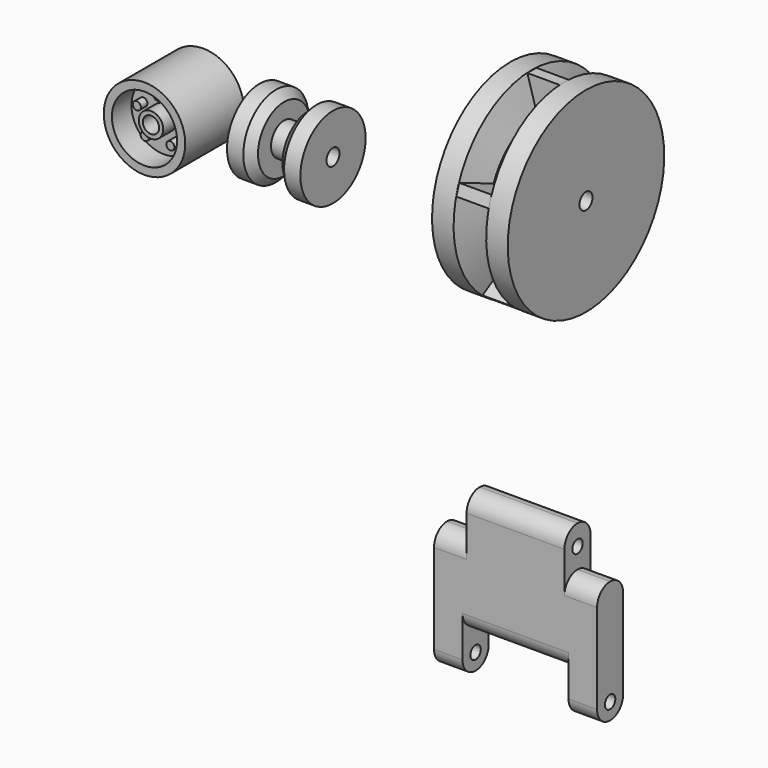
from build123d import *

# Parameters (mm, degrees)
F1_DEPTH  = 5.08
F2_R      = 1.016
F3_DEPTH  = 25.4
F4_R      = 2.53999
F5_R      = 1.016
F6_DEPTH  = 25.4
F8_W      = 2.032
F8_H      = 3.6169881774
F8_H_2    = 1.4630118226
F9_DEPTH  = 2.54
F9_TAPER  = 8
F12_R     = 12.7
F12_R_2   = 3.81
F13_DEPTH = 2.54
F12_R_3   = 1.27
F14_DEPTH = 25.4
F15_R     = 1.27
F16_DEPTH = 2.54
F17_R     = 1.27
F19_DEPTH = 8.89
F20_R     = 6.35
F20_R_2   = 5.08
F21_DEPTH = 11.43
F20_R_3   = 0.635
F20_R_4   = 1.905
F22_DEPTH = 7.62
F23_DEPTH = 8.89
F20_R_5   = 1.27
F24_DEPTH = 10.16
F27_R     = 5.08
F27_R_2   = 0.7135199612
F27_R_3   = 2.286
F28_DEPTH = 2.6162
F27_R_4   = 1.27
F29_DEPTH = 25.4
F30_DEPTH = 1.27
F31_SIZE  = 1.27


# Not quite as in the source:
# - a fillet or chamfer is up to 0.001 mm smaller than in the source, because OpenCascade refuses the exact size


with BuildPart() as f1:
    # F0 (on Front) → F1 (new body)
    with BuildSketch(Plane.XZ):
        Polygon((7.62, 6.35), (0, 6.35), (-7.62, 6.35), (-7.62, 0), (-12.7, 0), (-12.7, -19.05), (-8.255, -19.05), (-8.255, -12.7), (0, -12.7), (8.255, -12.7), (8.255, -19.05), (12.7, -19.05), (12.7, 0), (7.62, 0), align=None)
    extrude(amount=F1_DEPTH)

    # F2 (on face) → F3 (cut)
    with BuildSketch(Plane(origin=(-7.62, 0, 0), x_dir=(0, -1, 0), z_dir=(-1, 0, 0))):
        with Locations((2.54, 3.175)):
            Circle(F2_R)
    extrude(amount=-F3_DEPTH, mode=Mode.SUBTRACT)

    # F4 (radius 2.54 in the source; OpenCascade refuses exactly that, so slightly less here)
    f4_edges = [f1.edges().sort_by_distance(p)[0] for p in [
        (0, -5.08, 6.35),
        (0, 0, 6.35),
        (-10.16, -5.08, 0),
        (-10.16, 0, 0),
        (10.16, -5.08, 0),
        (10.16, 0, 0),
        (10.4775, -5.08, -19.05),
        (10.4775, 0, -19.05),
        (-10.4775, 0, -19.05),
        (-10.4775, -5.08, -19.05),
        (0, -5.08, -12.7),
        (0, 0, -12.7),
    ]]
    fillet(f4_edges, radius=F4_R)

    # F5 (on face) → F6 (cut, symmetric)
    with BuildSketch(Plane.YZ.offset(-8.255)):
        with Locations((-2.54, -16.51)):
            Circle(F5_R)
    extrude(amount=F6_DEPTH, both=True, mode=Mode.SUBTRACT)

    # F8 (on face) → F9 (join)
    with BuildSketch(Plane(origin=(0, 0, 0), x_dir=(-1, 0, 0), z_dir=(0, 1, 0))):
        with Locations((0, 0.7315059113)):
            Rectangle(F8_W, F8_H)
        with Locations((0, -1.8084940887)):
            Rectangle(F8_W, F8_H_2)
    extrude(amount=F9_DEPTH, taper=F9_TAPER)


with BuildPart() as f11:
    # F10 (on Front) → F11 (revolve)
    with BuildSketch(Plane.XZ):
        Polygon((-4.8794146568, 64.516250478), (-4.8794146568, 49.276250478), (6.9114146568, 49.276250478), (6.9114146568, 64.516250478), (3.556, 64.516250478), (2.032, 59.436250478), (0, 59.436250478), (-1.524, 64.516250478), align=None)
    revolve(axis=Axis((1.016, 0, 49.276250478), (-1, 0, 0)))

    # F12 (on face) → F13 (cut)
    with BuildSketch(Plane(origin=(-4.8794146568, 0, 0), x_dir=(0, -1, 0), z_dir=(-1, 0, 0))):
        with Locations((0, 49.276250478)):
            Circle(F12_R)
        with Locations((0, 49.276250478)):
            Circle(F12_R_2, mode=Mode.SUBTRACT)
    extrude(amount=-F13_DEPTH, mode=Mode.SUBTRACT)

    # F12 (on face) → F14 (cut)
    with BuildSketch(Plane(origin=(-4.8794146568, 0, 0), x_dir=(0, -1, 0), z_dir=(-1, 0, 0))):
        with Locations((0, 49.276250478)):
            Circle(F12_R_3)
    extrude(amount=-F14_DEPTH, mode=Mode.SUBTRACT)

    # F15 (on face) → F16 (join)
    with BuildSketch(Plane(origin=(-4.8794146568, 0, 0), x_dir=(0, -1, 0), z_dir=(-1, 0, 0))):
        with Locations((-7.0360511637, 53.3382660334)):
            Circle(F15_R)
        with Locations((0, 57.4005320668)):
            Circle(F15_R)
        with Locations((7.0360511637, 53.3382660334)):
            Circle(F15_R)
        with Locations((-7.0360511637, 45.2137339666)):
            Circle(F15_R)
        with Locations((0, 41.1514679332)):
            Circle(F15_R)
        with Locations((7.0360511637, 45.2137339666)):
            Circle(F15_R)
    extrude(amount=-F16_DEPTH)

    # F17
    f17_edges = [f11.edges().sort_by_distance(p)[0] for p in [
        (-4.879415, 8.306051, 53.338266),
        (-4.879415, 8.306051, 45.213734),
        (-4.879415, 1.27, 41.151468),
        (-4.879415, -5.766051, 45.213734),
        (-4.879415, -5.766051, 53.338266),
        (-4.879415, 1.27, 57.400532),
    ]]
    fillet(f17_edges, radius=F17_R)

    # F18 (on face) → F19 (join)
    with BuildSketch(Plane.YZ.offset(6.9114146568)):
        Polygon((0.8676911239, 64.4520207786), (-0.887604639, 64.4520207786), (-0.9478044813, 57.1678504348), (0.8676911239, 57.1678504348), align=None)
        Polygon((-14.164883931, 54.7910447011), (-14.7073001519, 53.1216592278), (-7.7982452549, 50.8134733494), (-7.2372262597, 52.540112275), align=None)
        Polygon((-9.6220708399, 37.5088104483), (-8.2020067376, 36.4770734854), (-3.8717761389, 42.3347065041), (-5.3405429366, 43.4018280464), align=None)
        Polygon((8.2181171098, 36.488778356), (9.6381812121, 37.5205153188), (5.4053560043, 43.4489174963), (3.9365892065, 42.3817959541), align=None)
        Polygon((14.7011465373, 53.1405981062), (14.1587303164, 54.8099835795), (7.2124698708, 52.6163046055), (7.773488866, 50.88966568), align=None)
    extrude(amount=-F19_DEPTH)


with BuildPart() as f21:
    # F20 (on Front) → F21 (new body)
    with BuildSketch(Plane.XZ):
        with Locations((-52.7230575681, 44.4563888013)):
            Circle(F20_R)
        with Locations((-52.7230575681, 44.4563888013)):
            Circle(F20_R_2, mode=Mode.SUBTRACT)
    extrude(amount=F21_DEPTH)

    # F20 (on Front) → F22 (join)
    with BuildSketch(Plane.XZ):
        with Locations((-52.7230575681, 44.4563888013)):
            Circle(F20_R_2)
        with Locations((-54.7188482534, 41.709418585)):
            Circle(F20_R_3, mode=Mode.SUBTRACT)
        with Locations((-50.7272668827, 41.709418585)):
            Circle(F20_R_3, mode=Mode.SUBTRACT)
        with Locations((-55.9523147314, 45.5056380579)):
            Circle(F20_R_3, mode=Mode.SUBTRACT)
        with Locations((-52.7230575681, 44.4563888013)):
            Circle(F20_R_4, mode=Mode.SUBTRACT)
        with Locations((-49.4938004048, 45.5056380579)):
            Circle(F20_R_3, mode=Mode.SUBTRACT)
        with Locations((-52.7230575681, 47.8518307209)):
            Circle(F20_R_3, mode=Mode.SUBTRACT)
    extrude(amount=F22_DEPTH)

    # F20 (on Front) → F23 (join)
    with BuildSketch(Plane.XZ):
        with Locations((-52.7230575681, 47.8518307209)):
            Circle(F20_R_3)
        with Locations((-55.9523147314, 45.5056380579)):
            Circle(F20_R_3)
        with Locations((-54.7188482534, 41.709418585)):
            Circle(F20_R_3)
        with Locations((-50.7272668827, 41.709418585)):
            Circle(F20_R_3)
        with Locations((-49.4938004048, 45.5056380579)):
            Circle(F20_R_3)
    extrude(amount=F23_DEPTH)

    # F20 (on Front) → F24 (join)
    with BuildSketch(Plane.XZ):
        with Locations((-52.7230575681, 44.4563888013)):
            Circle(F20_R_4)
        with Locations((-52.7230575681, 44.4563888013)):
            Circle(F20_R_5, mode=Mode.SUBTRACT)
    extrude(amount=F24_DEPTH)


with BuildPart() as f26:
    # F25 (on Front) → F26 (revolve)
    with BuildSketch(Plane.XZ):
        Polygon((-43.9292184118, 48.8412834392), (-43.9292184118, 43.7269604878), (-43.9292184118, 42.4912834392), (-32.4992184118, 42.4912834392), (-32.4992184118, 48.8412834392), (-36.3092184118, 48.8412834392), (-36.3092184118, 45.0312834392), (-40.1192184118, 45.0312834392), (-40.1192184118, 48.8412834392), align=None)
    revolve(axis=Axis((-38.2142184118, 0, 42.4912834392), (-1, 0, 0)))

    # F27 (on face) → F28 (cut)
    with BuildSketch(Plane(origin=(-43.9292184118, 0, 0), x_dir=(0, -1, 0), z_dir=(-1, 0, 0))):
        with Locations((0, 42.4912834392)):
            Circle(F27_R)
        with Locations((-3.4223097618, 41.379307591)):
            Circle(F27_R_2, mode=Mode.SUBTRACT)
        with Locations((0, 38.8928540051)):
            Circle(F27_R_2, mode=Mode.SUBTRACT)
        with Locations((3.4223097618, 41.379307591)):
            Circle(F27_R_2, mode=Mode.SUBTRACT)
        with Locations((-2.1151037528, 45.4024740045)):
            Circle(F27_R_2, mode=Mode.SUBTRACT)
        with Locations((0, 42.4912834392)):
            Circle(F27_R_3, mode=Mode.SUBTRACT)
        with Locations((2.1151037528, 45.4024740045)):
            Circle(F27_R_2, mode=Mode.SUBTRACT)
    extrude(amount=-F28_DEPTH, mode=Mode.SUBTRACT)

    # F27 (on face) → F29 (cut)
    with BuildSketch(Plane(origin=(-43.9292184118, 0, 0), x_dir=(0, -1, 0), z_dir=(-1, 0, 0))):
        with Locations((0, 42.4912834392)):
            Circle(F27_R_4)
    extrude(amount=-F29_DEPTH, mode=Mode.SUBTRACT)

    # F27 (on face) → F30 (cut)
    with BuildSketch(Plane(origin=(-43.9292184118, 0, 0), x_dir=(0, -1, 0), z_dir=(-1, 0, 0))):
        with Locations((-2.1151037528, 45.4024740045)):
            Circle(F27_R_2)
        with Locations((-3.4223097618, 41.379307591)):
            Circle(F27_R_2)
        with Locations((0, 38.8928540051)):
            Circle(F27_R_2)
        with Locations((3.4223097618, 41.379307591)):
            Circle(F27_R_2)
        with Locations((2.1151037528, 45.4024740045)):
            Circle(F27_R_2)
    extrude(amount=-F30_DEPTH, mode=Mode.SUBTRACT)

    # F31
    f31_edges = [f26.edges().sort_by_distance(p)[0] for p in [
        (-40.119218, 0, 36.141283),
        (-36.309218, 0, 36.141283),
    ]]
    chamfer(f31_edges, length=F31_SIZE)


solid = Compound([f1.part, f11.part, f21.part, f26.part])
